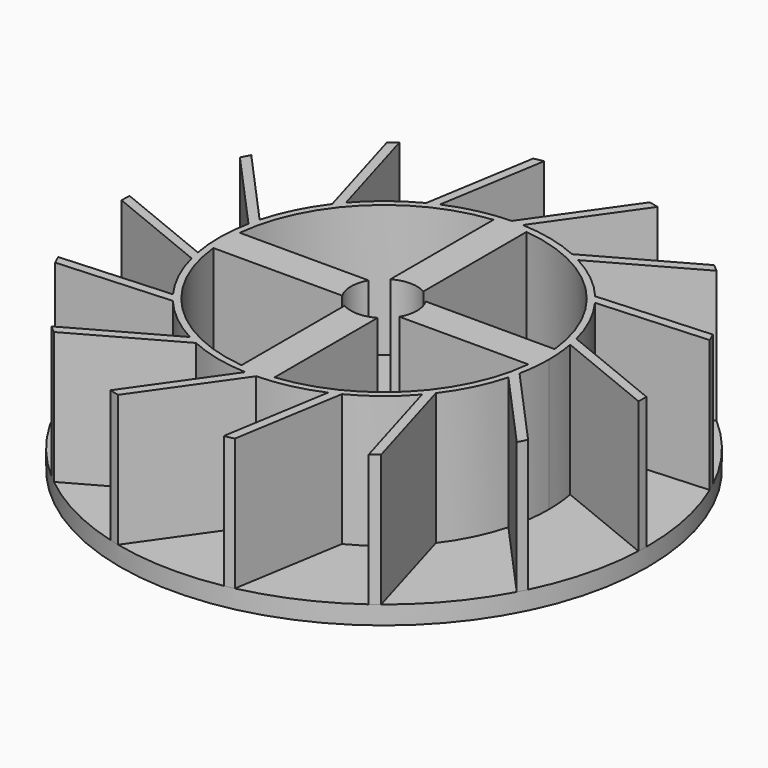
from build123d import *

# Parameters (mm, degrees)
F0_R     = 20
F1_DEPTH = 1.4
F3_DEPTH = 10
F4_DEPTH = 10
F5_DEPTH = 25.4
F6_DEPTH = 10


# Not quite as in the source:
# - after a boolean that leaves OpenCascade's solid faulty, fix() repairs it


with BuildPart() as f1:
    # F0 (on Top) → F1 (new body)
    with BuildSketch(Plane.XY):
        Circle(F0_R)
    extrude(amount=F1_DEPTH)

    # F2 (on face) → F3 (join)
    with BuildSketch(Plane.XY.offset(1.4)):
        with BuildLine():
            ThreePointArc((-5.7035176523, 11.1229441422), (-5.3278826262, 11.3076817572), (-4.9462725406, 11.4797381483))
            Line((-4.9462725406, 11.4797381483), (-3.5956301682, 19.6741313326))
            ThreePointArc((-3.5956301682, 19.6741313326), (-3.9575397764, 19.6045372023), (-4.3181055831, 19.528286258))
            Line((-4.3181055831, 19.528286258), (-5.7035176523, 11.1229441422))
        make_face()
        with BuildLine():
            ThreePointArc((-0.3126272478, 12.4960899566), (0.1059628635, 12.4995508668), (0.5244341406, 12.4889939079))
            Line((0.5244341406, 12.4889939079), (5.2967348245, 19.2858652956))
            ThreePointArc((5.2967348245, 19.2858652956), (4.940469773, 19.3801898448), (4.5825271615, 19.4679337582))
            Line((4.5825271615, 19.4679337582), (-0.3126272478, 12.4960899566))
        make_face()
        with BuildLine():
            ThreePointArc((5.1401828172, 11.3942319007), (5.5188211085, 11.2157306303), (5.8912702085, 11.0246512566))
            Line((5.8912702085, 11.0246512566), (13.140016525, 15.0777971111))
            ThreePointArc((13.140016525, 15.0777971111), (12.859958693, 15.3173582061), (12.5755342007, 15.5517182191))
            Line((12.5755342007, 15.5517182191), (5.1401828172, 11.3942319007))
        make_face()
        with BuildLine():
            ThreePointArc((9.574916635, 8.0356064757), (9.8386091491, 7.7104973906), (10.09126796, 7.3767412155))
            Line((10.09126796, 7.3767412155), (18.3807568009, 7.8833862917))
            ThreePointArc((18.3807568009, 7.8833862917), (18.2323750768, 8.2207359196), (18.0778024627, 8.5552941574))
            Line((18.0778024627, 8.5552941574), (9.574916635, 8.0356064757))
        make_face()
        with BuildLine():
            ThreePointArc((12.1132207847, 3.085430638), (12.2097399851, 2.6781055797), (12.2925663307, 2.2677771068))
            Line((12.2925663307, 2.2677771068), (19.9809627673, -0.8724258661))
            ThreePointArc((19.9809627673, -0.8724258661), (19.9936459712, -0.5041039365), (19.9995402372, -0.135610836))
            Line((19.9995402372, -0.135610836), (12.1132207847, 3.085430638))
        make_face()
        with BuildLine():
            Line((17.9601237896, -8.7996564401), (12.252352999, -2.4758525779))
            ThreePointArc((12.252352999, -2.4758525779), (12.1625820744, -2.8847178862), (12.0591711811, -3.2903480703))
            Line((12.0591711811, -3.2903480703), (17.6236940072, -9.4554433816))
            ThreePointArc((17.6236940072, -9.4554433816), (17.794930075, -9.1290998255), (17.9601237896, -8.7996564401))
        make_face()
        with BuildLine():
            Line((12.3634845589, -15.7208221656), (9.9647564366, -7.5467628264))
            ThreePointArc((9.9647564366, -7.5467628264), (9.7064756196, -7.8761875959), (9.4373092832, -8.1967794587))
            Line((9.4373092832, -8.1967794587), (11.7758365085, -16.1656943719))
            ThreePointArc((11.7758365085, -16.1656943719), (12.071710037, -15.9459655331), (12.3634845589, -15.7208221656))
        make_face()
        with BuildLine():
            Line((4.3181055831, -19.528286258), (5.7035176523, -11.1229441422))
            ThreePointArc((5.7035176523, -11.1229441422), (5.3278826262, -11.3076817572), (4.9462725406, -11.4797381483))
            Line((4.9462725406, -11.4797381483), (3.5956301682, -19.6741313326))
            ThreePointArc((3.5956301682, -19.6741313326), (3.9575397764, -19.6045372023), (4.3181055831, -19.528286258))
        make_face()
        with BuildLine():
            Line((-4.5825271615, -19.4679337582), (0.3126272478, -12.4960899566))
            ThreePointArc((0.3126272478, -12.4960899566), (-0.1059628635, -12.4995508668), (-0.5244341406, -12.4889939079))
            Line((-0.5244341406, -12.4889939079), (-5.2967348245, -19.2858652956))
            ThreePointArc((-5.2967348245, -19.2858652956), (-4.940469773, -19.3801898448), (-4.5825271615, -19.4679337582))
        make_face()
        with BuildLine():
            Line((-12.5755342007, -15.5517182191), (-5.1401828172, -11.3942319007))
            ThreePointArc((-5.1401828172, -11.3942319007), (-5.5188211085, -11.2157306303), (-5.8912702085, -11.0246512566))
            Line((-5.8912702085, -11.0246512566), (-13.140016525, -15.0777971111))
            ThreePointArc((-13.140016525, -15.0777971111), (-12.859958693, -15.3173582061), (-12.5755342007, -15.5517182191))
        make_face()
        with BuildLine():
            Line((-18.0778024627, -8.5552941574), (-9.574916635, -8.0356064757))
            ThreePointArc((-9.574916635, -8.0356064757), (-9.8386091491, -7.7104973906), (-10.09126796, -7.3767412155))
            Line((-10.09126796, -7.3767412155), (-18.3807568009, -7.8833862917))
            ThreePointArc((-18.3807568009, -7.8833862917), (-18.2323750768, -8.2207359196), (-18.0778024627, -8.5552941574))
        make_face()
        with BuildLine():
            Line((-19.9995402372, 0.135610836), (-12.1132207847, -3.085430638))
            ThreePointArc((-12.1132207847, -3.085430638), (-12.2097399851, -2.6781055797), (-12.2925663307, -2.2677771068))
            Line((-12.2925663307, -2.2677771068), (-19.9809627673, 0.8724258661))
            ThreePointArc((-19.9809627673, 0.8724258661), (-19.9936459712, 0.5041039365), (-19.9995402372, 0.135610836))
        make_face()
        with BuildLine():
            ThreePointArc((-12.252352999, 2.4758525779), (-12.1625820744, 2.8847178862), (-12.0591711811, 3.2903480703))
            Line((-12.0591711811, 3.2903480703), (-17.6236940072, 9.4554433816))
            ThreePointArc((-17.6236940072, 9.4554433816), (-17.794930075, 9.1290998255), (-17.9601237896, 8.7996564401))
            Line((-17.9601237896, 8.7996564401), (-12.252352999, 2.4758525779))
        make_face()
        with BuildLine():
            ThreePointArc((-9.9647564366, 7.5467628264), (-9.7064756196, 7.8761875959), (-9.4373092832, 8.1967794587))
            Line((-9.4373092832, 8.1967794587), (-11.7758365085, 16.1656943719))
            ThreePointArc((-11.7758365085, 16.1656943719), (-12.071710037, 15.9459655331), (-12.3634845589, 15.7208221656))
            Line((-12.3634845589, 15.7208221656), (-9.9647564366, 7.5467628264))
        make_face()
    extrude(amount=F3_DEPTH)

    # F2 (on face) → F4 (join)
    with BuildSketch(Plane.XY.offset(1.4)):
        with BuildLine():
            ThreePointArc((12.252352999, -2.4758525779), (12.437934163, -1.2441035954), (12.5, 0))
            ThreePointArc((12.5, 0), (12.4480335622, 1.1386221644), (12.2925663307, 2.2677771068))
            ThreePointArc((12.2925663307, 2.2677771068), (12.2097399851, 2.6781055797), (12.1132207847, 3.085430638))
            ThreePointArc((12.1132207847, 3.085430638), (11.3076817572, 5.3278826262), (10.09126796, 7.3767412155))
            ThreePointArc((10.09126796, 7.3767412155), (9.8386091491, 7.7104973906), (9.574916635, 8.0356064757))
            ThreePointArc((9.574916635, 8.0356064757), (7.8761875959, 9.7064756196), (5.8912702085, 11.0246512566))
            ThreePointArc((5.8912702085, 11.0246512566), (5.5188211085, 11.2157306303), (5.1401828172, 11.3942319007))
            ThreePointArc((5.1401828172, 11.3942319007), (2.8847178862, 12.1625820744), (0.5244341406, 12.4889939079))
            ThreePointArc((0.5244341406, 12.4889939079), (0.1059628635, 12.4995508668), (-0.3126272478, 12.4960899566))
            ThreePointArc((-0.3126272478, 12.4960899566), (-2.6781055797, 12.2097399851), (-4.9462725406, 11.4797381483))
            ThreePointArc((-4.9462725406, 11.4797381483), (-5.3278826262, 11.3076817572), (-5.7035176523, 11.1229441422))
            ThreePointArc((-5.7035176523, 11.1229441422), (-7.7104973906, 9.8386091491), (-9.4373092832, 8.1967794587))
            ThreePointArc((-9.4373092832, 8.1967794587), (-9.7064756196, 7.8761875959), (-9.9647564366, 7.5467628264))
            ThreePointArc((-9.9647564366, 7.5467628264), (-11.2157306303, 5.5188211085), (-12.0591711811, 3.2903480703))
            ThreePointArc((-12.0591711811, 3.2903480703), (-12.1625820744, 2.8847178862), (-12.252352999, 2.4758525779))
            ThreePointArc((-12.252352999, 2.4758525779), (-12.4995508668, 0.1059628635), (-12.2925663307, -2.2677771068))
            ThreePointArc((-12.2925663307, -2.2677771068), (-12.2097399851, -2.6781055797), (-12.1132207847, -3.085430638))
            ThreePointArc((-12.1132207847, -3.085430638), (-11.3076817572, -5.3278826262), (-10.09126796, -7.3767412155))
            ThreePointArc((-10.09126796, -7.3767412155), (-9.8386091491, -7.7104973906), (-9.574916635, -8.0356064757))
            ThreePointArc((-9.574916635, -8.0356064757), (-7.8761875959, -9.7064756196), (-5.8912702085, -11.0246512566))
            ThreePointArc((-5.8912702085, -11.0246512566), (-5.5188211085, -11.2157306303), (-5.1401828172, -11.3942319007))
            ThreePointArc((-5.1401828172, -11.3942319007), (-2.8847178862, -12.1625820744), (-0.5244341406, -12.4889939079))
            ThreePointArc((-0.5244341406, -12.4889939079), (-0.1059628635, -12.4995508668), (0.3126272478, -12.4960899566))
            ThreePointArc((0.3126272478, -12.4960899566), (2.6781055797, -12.2097399851), (4.9462725406, -11.4797381483))
            ThreePointArc((4.9462725406, -11.4797381483), (5.3278826262, -11.3076817572), (5.7035176523, -11.1229441422))
            ThreePointArc((5.7035176523, -11.1229441422), (7.7104973906, -9.8386091491), (9.4373092832, -8.1967794587))
            ThreePointArc((9.4373092832, -8.1967794587), (9.7064756196, -7.8761875959), (9.9647564366, -7.5467628264))
            ThreePointArc((9.9647564366, -7.5467628264), (11.2157306303, -5.5188211085), (12.0591711811, -3.2903480703))
            ThreePointArc((12.0591711811, -3.2903480703), (12.1625820744, -2.8847178862), (12.252352999, -2.4758525779))
        make_face()
        with BuildLine():
            ThreePointArc((11.9347182623, 1.25), (11.9836684523, 0.6258517607), (12, 0))
            ThreePointArc((12, 0), (11.9836684523, -0.6258517607), (11.9347182623, -1.25))
            ThreePointArc((11.9347182623, -1.25), (8.4852813742, -8.4852813742), (1.25, -11.9347182623))
            ThreePointArc((1.25, -11.9347182623), (0, -12), (-1.25, -11.9347182623))
            ThreePointArc((-1.25, -11.9347182623), (-8.4852813742, -8.4852813742), (-11.9347182623, -1.25))
            ThreePointArc((-11.9347182623, -1.25), (-12, 0), (-11.9347182623, 1.25))
            ThreePointArc((-11.9347182623, 1.25), (-8.4852813742, 8.4852813742), (-1.25, 11.9347182623))
            ThreePointArc((-1.25, 11.9347182623), (0, 12), (1.25, 11.9347182623))
            ThreePointArc((1.25, 11.9347182623), (8.4852813742, 8.4852813742), (11.9347182623, 1.25))
        make_face(mode=Mode.SUBTRACT)
    extrude(amount=F4_DEPTH)

    # F2 (on face) → F5 (cut)
    with BuildSketch(Plane.XY.offset(1.4)):
        with BuildLine():
            ThreePointArc((2.5, 0), (2.4148145657, 0.6470476128), (2.1650635095, 1.25))
            ThreePointArc((2.1650635095, 1.25), (1.767766953, 1.767766953), (1.25, 2.1650635095))
            ThreePointArc((1.25, 2.1650635095), (0, 2.5), (-1.25, 2.1650635095))
            ThreePointArc((-1.25, 2.1650635095), (-1.767766953, 1.767766953), (-2.1650635095, 1.25))
            ThreePointArc((-2.1650635095, 1.25), (-2.5, 0), (-2.1650635095, -1.25))
            ThreePointArc((-2.1650635095, -1.25), (-1.767766953, -1.767766953), (-1.25, -2.1650635095))
            ThreePointArc((-1.25, -2.1650635095), (0, -2.5), (1.25, -2.1650635095))
            ThreePointArc((1.25, -2.1650635095), (1.767766953, -1.767766953), (2.1650635095, -1.25))
            ThreePointArc((2.1650635095, -1.25), (2.4148145657, -0.6470476128), (2.5, 0))
        make_face()
    extrude(amount=-F5_DEPTH, mode=Mode.SUBTRACT)

    # F2 (on face) → F6 (join)
    with BuildSketch(Plane.XY.offset(1.4)):
        with BuildLine():
            Line((1.25, 2.1650635095), (1.25, 11.9347182623))
            ThreePointArc((1.25, 11.9347182623), (0, 12), (-1.25, 11.9347182623))
            Line((-1.25, 11.9347182623), (-1.25, 2.1650635095))
            ThreePointArc((-1.25, 2.1650635095), (0, 2.5), (1.25, 2.1650635095))
        make_face()
        with BuildLine():
            ThreePointArc((11.9347182623, -1.25), (11.9836684523, -0.6258517607), (12, 0))
            ThreePointArc((12, 0), (11.9836684523, 0.6258517607), (11.9347182623, 1.25))
            Line((11.9347182623, 1.25), (2.1650635095, 1.25))
            ThreePointArc((2.1650635095, 1.25), (2.4148145657, 0.6470476128), (2.5, 0))
            ThreePointArc((2.5, 0), (2.4148145657, -0.6470476128), (2.1650635095, -1.25))
            Line((2.1650635095, -1.25), (11.9347182623, -1.25))
        make_face()
        with BuildLine():
            ThreePointArc((-1.25, -11.9347182623), (0, -12), (1.25, -11.9347182623))
            Line((1.25, -11.9347182623), (1.25, -2.1650635095))
            ThreePointArc((1.25, -2.1650635095), (0, -2.5), (-1.25, -2.1650635095))
            Line((-1.25, -2.1650635095), (-1.25, -11.9347182623))
        make_face()
        with BuildLine():
            Line((-2.1650635095, 1.25), (-11.9347182623, 1.25))
            ThreePointArc((-11.9347182623, 1.25), (-12, 0), (-11.9347182623, -1.25))
            Line((-11.9347182623, -1.25), (-2.1650635095, -1.25))
            ThreePointArc((-2.1650635095, -1.25), (-2.5, 0), (-2.1650635095, 1.25))
        make_face()
    extrude(amount=F6_DEPTH)

    add(f1.part.fix(), mode=Mode.REPLACE)


solid = f1.part
